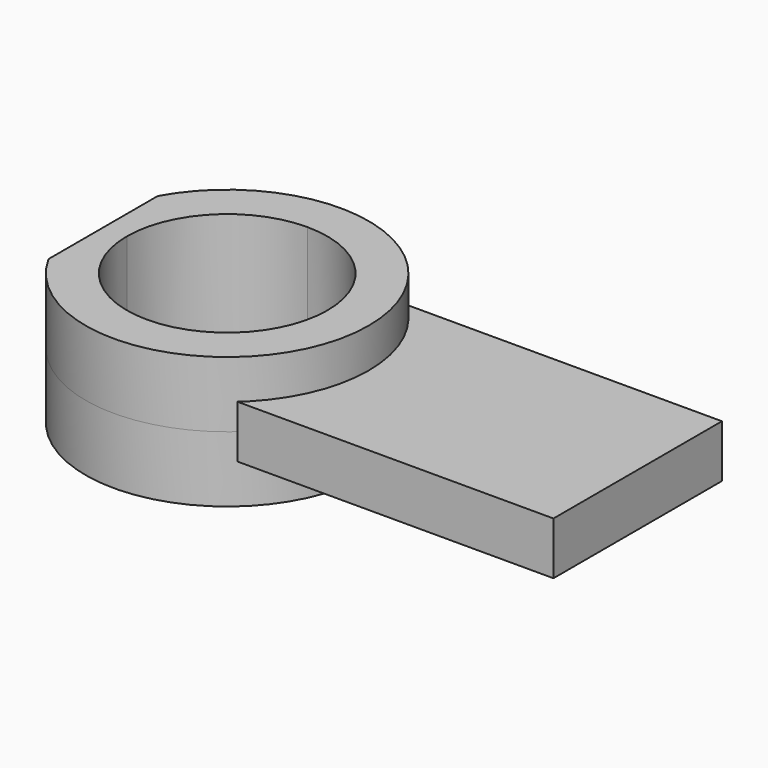
from build123d import *

# Parameters (mm, degrees)
F1_DEPTH      = 25
F1_DEPTH_BACK = 25
F2_DEPTH      = 10
F2_DEPTH_BACK = 10
F4_DEPTH      = 40


with BuildPart() as f1:
    # F0 (on Top) → F1 (new body, two sides)
    with BuildSketch(Plane.XY) as f1_sk:
        with BuildLine():
            ThreePointArc((-83.0851361962, 14.0932304172), (-44.9472909192, -13.0255649041), (0, 0))
            Line((0, 0), (0, 80))
            ThreePointArc((0, 80), (-44.9472909192, 93.0255649041), (-83.0851361962, 65.9067695828))
            Line((-83.0851361962, 65.9067695828), (-83.0851361962, 14.0932304172))
        make_face()
        with BuildLine():
            Line((0, 80), (0, 0))
            ThreePointArc((0, 0), (13.1707529219, 18.1030103156), (17.8301045695, 40))
            ThreePointArc((17.8301045695, 40), (13.1707529219, 61.8969896844), (0, 80))
        make_face()
    extrude(amount=F1_DEPTH)
    extrude(f1_sk.sketch, amount=-F1_DEPTH_BACK)

    # F3 (on face) → F4 (cut)
    with BuildSketch(Plane.XY.offset(25)):
        with BuildLine():
            ThreePointArc((2.1356884389, 40), (-9.0201962122, 66.9326880249), (-35.952884237, 78.0885726759))
            Line((-35.952884237, 78.0885726759), (-35.952884237, 40))
            Line((-35.952884237, 40), (2.1356884389, 40))
        make_face()
        with BuildLine():
            Line((-35.952884237, 40), (-35.952884237, 78.0885726759))
            ThreePointArc((-35.952884237, 78.0885726759), (-62.8855722619, 66.9326880249), (-74.0414569129, 40))
            Line((-74.0414569129, 40), (-35.952884237, 40))
        make_face()
        with BuildLine():
            Line((2.1356884389, 40), (-35.952884237, 40))
            Line((-35.952884237, 40), (-35.952884237, 1.9114273241))
            ThreePointArc((-35.952884237, 1.9114273241), (-9.0201962122, 13.0673119751), (2.1356884389, 40))
        make_face()
        with BuildLine():
            Line((-35.952884237, 1.9114273241), (-35.952884237, 40))
            Line((-35.952884237, 40), (-74.0414569129, 40))
            ThreePointArc((-74.0414569129, 40), (-62.8855722619, 13.0673119751), (-35.952884237, 1.9114273241))
        make_face()
    extrude(amount=-F4_DEPTH, mode=Mode.SUBTRACT)


with BuildPart() as f2:
    # F0 (on Top) → F2 (new body, two sides)
    with BuildSketch(Plane.XY) as f2_sk:
        with BuildLine():
            ThreePointArc((17.8301045695, 40), (13.1707529219, 18.1030103156), (0, 0))
            Line((0, 0), (120, 0))
            Line((120, 0), (120, 80))
            Line((120, 80), (0, 80))
            ThreePointArc((0, 80), (13.1707529219, 61.8969896844), (17.8301045695, 40))
        make_face()
        with BuildLine():
            Line((0, 80), (0, 0))
            ThreePointArc((0, 0), (13.1707529219, 18.1030103156), (17.8301045695, 40))
            ThreePointArc((17.8301045695, 40), (13.1707529219, 61.8969896844), (0, 80))
        make_face()
    extrude(amount=F2_DEPTH)
    extrude(f2_sk.sketch, amount=-F2_DEPTH_BACK)


solid = Compound([f1.part, f2.part])
